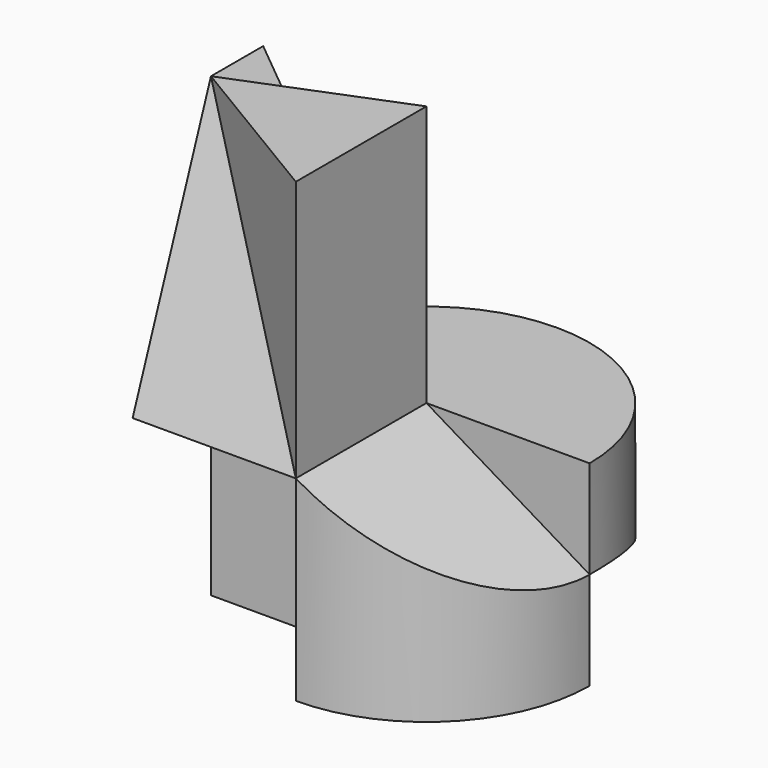
from build123d import *

# Parameters (mm, degrees)
F0_W      = 100
F0_H      = 100
F1_DEPTH  = 140
F3_DEPTH  = 140.001
F5_DEPTH  = 80
F9_DEPTH  = 50.00099999
F11_DEPTH = 50.00099999
F6_W      = 50
F6_H      = 80
F14_W     = 30
F14_H     = 60
F16_DEPTH = 49.99


with BuildPart() as f1:
    # F0 (on Top) → F1 (new body)
    with BuildSketch(Plane.XY):
        with Locations((50, 50)):
            Rectangle(F0_W, F0_H)
    extrude(amount=F1_DEPTH)

    # F2 (on face) → F3 (cut, through all)
    with BuildSketch(Plane.XY.offset(140)):
        with BuildLine():
            ThreePointArc((0, 50), (14.6446609407, 85.3553390593), (50, 100))
            Line((50, 100), (0, 100))
            Line((0, 100), (0, 50))
        make_face()
        with BuildLine():
            ThreePointArc((50, 100), (85.3553390593, 85.3553390593), (100, 50))
            Line((100, 50), (100, 100))
            Line((100, 100), (50, 100))
        make_face()
        with BuildLine():
            Line((100, 0), (100, 50))
            ThreePointArc((100, 50), (85.3553390593, 14.6446609407), (50, 0))
            Line((50, 0), (100, 0))
        make_face()
    extrude(amount=-F3_DEPTH, mode=Mode.SUBTRACT)

    # F4 (on face) → F5 (cut)
    with BuildSketch(Plane.XY.offset(140)):
        with BuildLine():
            ThreePointArc((100, 50), (50, 100), (0, 50))
            Line((0, 50), (50, 50))
            Line((50, 50), (50, 0))
            ThreePointArc((50, 0), (85.3553390593, 14.6446609407), (100, 50))
        make_face()
    extrude(amount=-F5_DEPTH, mode=Mode.SUBTRACT)

    # F8 (on face) → F9 (cut, through all)
    with BuildSketch(Plane.XZ.offset(-50)):
        Polygon((100, 60), (50.001, 60), (100, 30), align=None)
    extrude(amount=F9_DEPTH, mode=Mode.SUBTRACT)

    # F10 (on face) → F11 (cut, through all)
    with BuildSketch(Plane.XZ.offset(-50)):
        Polygon((50.001, 0), (100, 0), (100, 29.99), align=None)
    extrude(amount=-F11_DEPTH, mode=Mode.SUBTRACT)

    # F6 (on face) → F13 section 0
    with BuildSketch(Plane.XZ, mode=Mode.PRIVATE) as f13_s0:
        with Locations((25, 100)):
            Rectangle(F6_W, F6_H)
    loft([f13_s0.sketch, Vertex(0, 30, 140)], mode=Mode.SUBTRACT)

    # F14 (on face) → F16 (cut)
    with BuildSketch(Plane(origin=(0, 0, 0), x_dir=(0, -1, 0), z_dir=(-1, 0, 0))):
        with Locations((-15, 30)):
            Rectangle(F14_W, F14_H)
    extrude(amount=-F16_DEPTH, mode=Mode.SUBTRACT)

    # F17 (on face) → F18 section 0
    with BuildSketch(Plane.XY.offset(140), mode=Mode.PRIVATE) as f18_s0:
        Polygon((0, 50), (0, 30), (50, 50), align=None)
    loft([f18_s0.sketch, Vertex(50, 50, 60)], mode=Mode.SUBTRACT)


solid = f1.part
